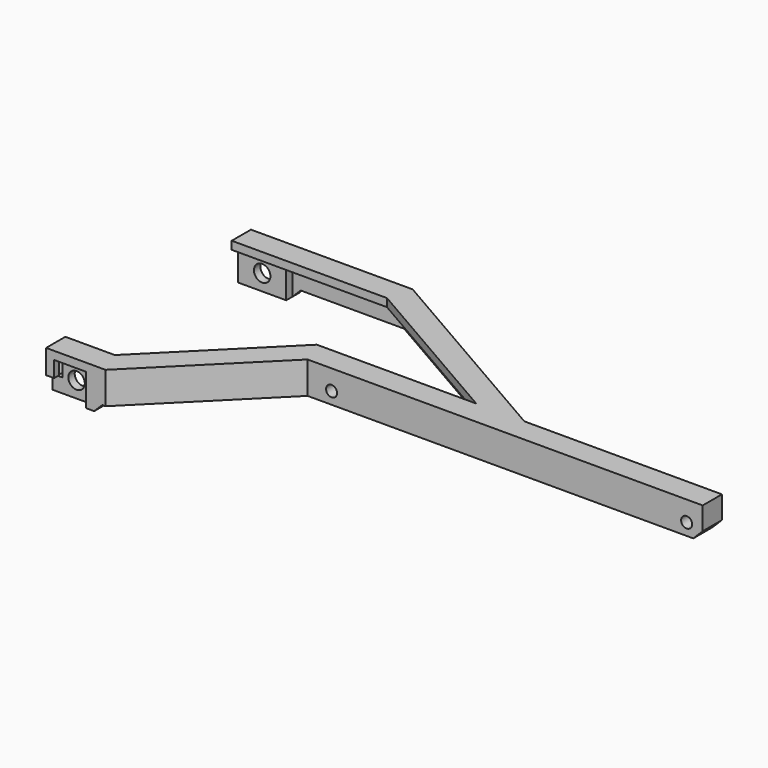
from build123d import *

# Parameters (mm, degrees)
F1_DEPTH      = 1.5875
F3_DEPTH      = 4.7625
F4_W          = 6.35
F4_H          = 6.35
F4_W_2        = 4.7625
F4_H_2        = 4.7625
F5_DEPTH      = 3.175
F6_SIZE       = 1.8598642
F7_W          = 28.575
F7_H          = 3.175
F8_DEPTH      = 1.5875
F9_W          = 6.35
F9_H          = 1.5875
F10_DEPTH     = 6.35
F11_R         = 1.0922
F11_R_2       = 1.63322
F12_DEPTH     = 25.4
F13_SIZE      = 1.58749
F14_R         = 0.396875
F15_DEPTH     = 6.35
F16_R         = 1.63322
F17_DEPTH     = 1.5875
F18_W         = 141.7602359697
F18_H         = 50.7137336135
F19_DEPTH     = 7.9375
F20_W         = 1.5875
F20_H         = 3.175
F21_DEPTH     = 1.5875
F22_R         = 0.396875
F23_DEPTH     = 3.175
F24_T4_DEPTH  = 1.4175116858
F24_S5_R      = 0.396875
F24_T6_DEPTH  = 2
F24_T10_DEPTH = 1.4175116858
F24_S11_R     = 0.396875
F24_T12_DEPTH = 2
F24_T16_DEPTH = 2.8350233717
F24_S17_R     = 0.396875
F24_T18_DEPTH = 3


# Not quite as in the source:
# - a fillet or chamfer that OpenCascade refuses, or shapes differently, is made with other operations: its cross-section is extruded or revolved along the edge and cut away or added
# - a fillet or chamfer is up to 0.001 mm smaller than in the source, because OpenCascade refuses the exact size


with BuildPart() as f1:
    # F0 (on Top) → F1 (new body)
    with BuildSketch(Plane.XY):
        Polygon((-87.87765, 22.225), (-127, 22.225), (-127, 17.4625), (-48.7553, 17.4625), (-26.5303, -4.7625), (26.5303, -4.7625), (48.7553, 17.4625), (127, 17.4625), (127, 22.225), (87.87765, 22.225), (46.7826079092, 45.9512336135), (-46.7826079092, 45.9512336135), align=None)
        Polygon((-24.5576079092, 0), (-46.7826079092, 22.225), (-78.35265, 22.225), (-45.5064998802, 41.1887336135), (45.5064998802, 41.1887336135), (78.35265, 22.225), (46.7826079092, 22.225), (24.5576079092, 0), align=None, mode=Mode.SUBTRACT)
    extrude(amount=F1_DEPTH)

    # F2 (on face) → F3 (join)
    with BuildSketch(Plane(origin=(0, 0, 0), x_dir=(1, 0, 0), z_dir=(0, 0, -1))):
        Polygon((-48.7553, -17.4625), (-127, -17.4625), (-127, -19.05), (-93.376911314, -19.05), (-87.87765, -22.225), (-46.7826079092, -45.9512336135), (46.7826079092, -45.9512336135), (87.87765, -22.225), (93.376911314, -19.05), (127, -19.05), (127, -17.4625), (48.7553, -17.4625), (26.5303, 4.7625), (-26.5303, 4.7625), align=None)
        Polygon((-48.0977359697, -19.05), (-25.8727359697, 3.175), (-4.2897640303, 3.175), (-4.2897640303, 1.5875), (24.2852359697, 1.5875), (24.2852359697, 3.175), (25.8727359697, 3.175), (48.0977359697, -19.05), (90.201911314, -19.05), (46.3572385662, -44.3637336135), (24.2852359697, -44.3637336135), (24.2852359697, -42.7762336135), (-4.2897640303, -42.7762336135), (-4.2897640303, -44.3637336135), (-46.3572385662, -44.3637336135), (-90.201911314, -19.05), align=None, mode=Mode.SUBTRACT)
    extrude(amount=F3_DEPTH)

    # F4 (on face) → F5 (join, through all)
    with BuildSketch(Plane(origin=(0, 19.05, 0), x_dir=(-1, 0, 0), z_dir=(0, 1, 0))):
        with Locations((-53.5178, -1.5875)):
            Rectangle(F4_W, F4_H)
        with Locations((-123.825, -1.5875)):
            Rectangle(F4_W, F4_H)
        with Locations((124.61875, -2.38125)):
            Rectangle(F4_W_2, F4_H_2)
        with Locations((55.89905, -2.38125)):
            Rectangle(F4_W_2, F4_H_2)
    extrude(amount=F5_DEPTH)

    # F6
    f6_edges = [f1.edges().sort_by_distance(p)[0] for p in [
        (-127, 19.84375, -4.7625),
        (-122.2375, 20.6375, -4.7625),
        (-58.2803, 20.6375, -4.7625),
        (-53.5178, 20.6375, -4.7625),
        (50.3428, 20.6375, -4.7625),
        (56.6928, 20.6375, -4.7625),
        (120.65, 20.6375, -4.7625),
        (127, 19.84375, -4.7625),
    ]]
    chamfer(f6_edges, length=F6_SIZE)

    # F7 (on face) → F8 (join)
    with BuildSketch(Plane(origin=(0, 0, -4.7625), x_dir=(1, 0, 0), z_dir=(0, 0, -1))):
        with Locations((9.9977359697, 3.175)):
            Rectangle(F7_W, F7_H)
        with Locations((9.9977359697, -44.3637336135)):
            Rectangle(F7_W, F7_H)
    extrude(amount=F8_DEPTH)

    # F9 (on face) → F10 (cut, through all)
    with BuildSketch(Plane(origin=(0, 0, -6.35), x_dir=(1, 0, 0), z_dir=(0, 0, -1))):
        with Locations((19.5227359697, 3.96875)):
            Rectangle(F9_W, F9_H)
        with Locations((19.5227359697, -45.1574836135)):
            Rectangle(F9_W, F9_H)
    extrude(amount=-F10_DEPTH, mode=Mode.SUBTRACT)

    # F11 (on face) → F12 (cut, through all)
    with BuildSketch(Plane.XZ.offset(3.175)):
        with Locations((53.5178, -2.38125)):
            Circle(F11_R)
        with Locations((123.825, -2.38125)):
            Circle(F11_R)
        with Locations((-124.61875, -2.38125)):
            Circle(F11_R)
        with Locations((-55.89905, -2.38125)):
            Circle(F11_R)
        with Locations((19.5227359697, -3.175)):
            Circle(F11_R_2)
    extrude(amount=-F12_DEPTH, mode=Mode.SUBTRACT)

    # F13 (size 1.5875 in the source; OpenCascade refuses exactly that, so slightly less here)
    f13_edges = [f1.edges().sort_by_distance(p)[0] for p in [
        (-4.289764, -3.96875, -4.7625),
        (24.285236, -3.96875, -4.7625),
        (-4.289764, 45.157484, -4.7625),
        (24.285236, 45.157484, -4.7625),
    ]]
    chamfer(f13_edges, length=F13_SIZE)

    # F14 (on face) → F15 (cut, through all)
    with BuildSketch(Plane(origin=(0, 0, -6.35), x_dir=(1, 0, 0), z_dir=(0, 0, -1))):
        with Locations((22.6977359697, 3.175)):
            Circle(F14_R)
        with Locations((22.6977359697, -44.3637336135)):
            Circle(F14_R)
    extrude(amount=-F15_DEPTH, mode=Mode.SUBTRACT)

    # F16 (on face) → F17 (cut, through all)
    with BuildSketch(Plane(origin=(0, 44.3637336135, 0), x_dir=(-1, 0, 0), z_dir=(0, 1, 0))):
        with Locations((-19.5227359697, -3.175)):
            Circle(F16_R)
    extrude(amount=-F17_DEPTH, mode=Mode.SUBTRACT)

    # F18 (on face) → F19 (cut, through all)
    with BuildSketch(Plane(origin=(0, 0, -6.35), x_dir=(1, 0, 0), z_dir=(0, 0, -1))):
        with Locations((-56.1198820151, -20.5943668067)):
            Rectangle(F18_W, F18_H)
    extrude(amount=-F19_DEPTH, mode=Mode.SUBTRACT)

    # F20 (on face) → F21 (cut, through all)
    with BuildSketch(Plane.YZ.offset(16.3477359697)):
        with Locations((-3.96875, -4.7625)):
            Rectangle(F20_W, F20_H)
        with Locations((45.1574836135, -4.7625)):
            Rectangle(F20_W, F20_H)
    extrude(amount=-F21_DEPTH, mode=Mode.SUBTRACT)

    # F22 (on face) → F23 (cut, through all)
    with BuildSketch(Plane(origin=(0, 0, -3.175), x_dir=(1, 0, 0), z_dir=(0, 0, -1))):
        with Locations((16.3477359697, -44.3637336135)):
            Circle(F22_R)
        with Locations((16.3477359697, 3.175)):
            Circle(F22_R)
    extrude(amount=-F23_DEPTH, mode=Mode.SUBTRACT)

    # F24: chamfer of 0.396875 on 3 edges, made by hand


with BuildPart() as f24_tool2:
    # F24_s3 → F24_t4 (new body)
    with BuildSketch(Plane.YZ.offset(17.7652476556)):
        Polygon((-2.778125, -3.175), (-3.175, -3.571875), (-3.175, -3.175), align=None)
    extrude(amount=-F24_T4_DEPTH)

    # F24_s5 → F24_t6 (intersect, symmetric)
    with BuildSketch(Plane.XY.offset(-3.4)):
        with Locations((16.3477359697, -3.175)):
            Circle(F24_S5_R)
    extrude(amount=F24_T6_DEPTH, both=True, mode=Mode.INTERSECT)


with BuildPart() as f1_1:
    add(f1.part)

    # F24_t1: cut F24_tool2
    add(f24_tool2.part, mode=Mode.SUBTRACT)


with BuildPart() as f24_tool8:
    # F24_s9 → F24_t10 (new body)
    with BuildSketch(Plane.YZ.offset(16.3477359697)):
        Polygon((-2.778125, -3.175), (-3.175, -3.571875), (-3.175, -3.175), align=None)
    extrude(amount=-F24_T10_DEPTH)

    # F24_s11 → F24_t12 (intersect, symmetric)
    with BuildSketch(Plane.XY.offset(-3.4)):
        with Locations((16.3477359697, -3.175)):
            Circle(F24_S11_R)
    extrude(amount=F24_T12_DEPTH, both=True, mode=Mode.INTERSECT)


with BuildPart() as f1_2:
    add(f1_1.part)

    # F24_t7: cut F24_tool8
    add(f24_tool8.part, mode=Mode.SUBTRACT)


with BuildPart() as f24_tool14:
    # F24_s15 → F24_t16 (new body)
    with BuildSketch(Plane.YZ.offset(14.9302242839)):
        Polygon((44.3637336135, -3.571875), (43.9668586135, -3.175), (44.3637336135, -3.175), align=None)
    extrude(amount=F24_T16_DEPTH)

    # F24_s17 → F24_t18 (intersect, symmetric)
    with BuildSketch(Plane.XY.offset(-3.4)):
        with Locations((16.3477359697, 44.3637336135)):
            Circle(F24_S17_R)
    extrude(amount=F24_T18_DEPTH, both=True, mode=Mode.INTERSECT)


with BuildPart() as f1_3:
    add(f1_2.part)

    # F24_t13: cut F24_tool14
    add(f24_tool14.part, mode=Mode.SUBTRACT)


solid = f1_3.part
